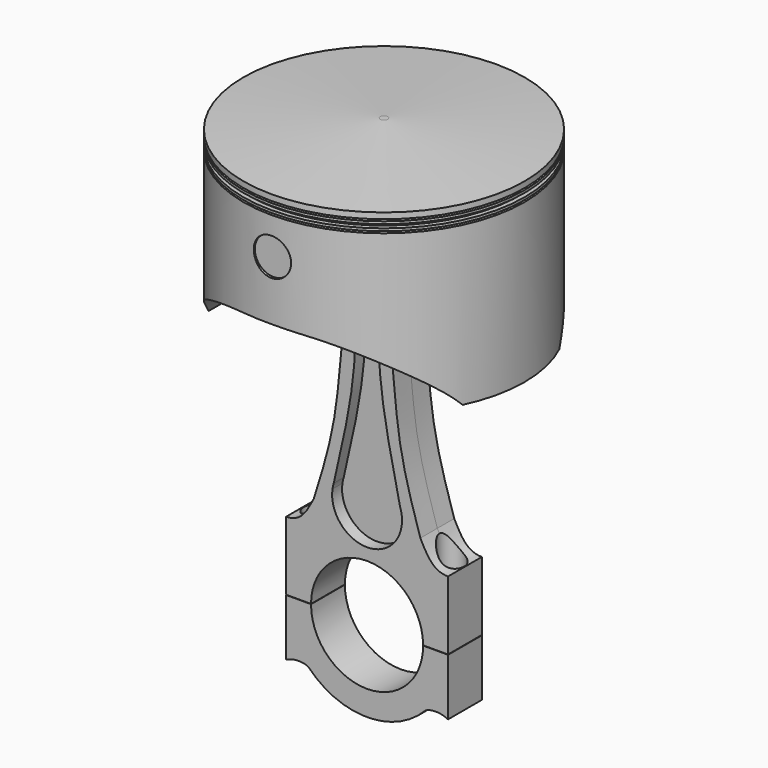
from build123d import *

# Parameters (mm, degrees)
F0_R           = 56.5
F1_DEPTH       = 75
F2_W           = 2
F2_H           = 0.75
F2_H_2         = 1.5
F4_SIZE2       = 4
F4_SIZE        = 55
F5_R           = 7.5
F6_DEPTH       = 100
F7_R           = 53.4676328736
F8_DEPTH       = 35.3
F10_END_RADIUS = 53.4676328736
F10_REACH      = 175.370336275
F11_END_RADIUS = 53.4676328736
F11_REACH      = 175.370336275
F12_W          = 30
F12_H          = 20
F13_DEPTH      = 65
F14_R          = 7.5
F15_DEPTH      = 8.5
F17_DEPTH      = 5
F19_DEPTH      = 5
F20_R          = 5
F21_DEPTH      = 95
F22_R          = 4
F23_DEPTH      = 12.5
F25_DEPTH      = 8.5
F26_R          = 4
F27_DEPTH      = 25
F28_R          = 7.5
F29_DEPTH      = 55.5


with BuildPart() as f1:
    # F0 (on Top) → F1 (new body)
    with BuildSketch(Plane.XY):
        Circle(F0_R)
    extrude(amount=F1_DEPTH)

    # F2 (on Front) → F3 (revolve, cut)
    with BuildSketch(Plane.XZ):
        with Locations((-55.6016643415, 68.2410276427)):
            Rectangle(F2_W, F2_H)
        with Locations((-55.6016643415, 66.1160276427)):
            Rectangle(F2_W, F2_H_2)
        with Locations((-55.6016643415, 63.9910276427)):
            Rectangle(F2_W, F2_H)
    revolve(axis=Axis((0, 0, 69.4315228611), (0, 0, 1)), mode=Mode.SUBTRACT)

    # F4
    f4_edges = [f1.edges().sort_by_distance(p)[0] for p in [
        (-56.5, 0, 75),
    ]]
    f4_side = f1.faces().sort_by_distance((0, 0, 75))[0]
    chamfer(f4_edges, length=F4_SIZE, length2=F4_SIZE2, reference=f4_side)

    # F5 (on Front) → F6 (cut, symmetric)
    with BuildSketch(Plane.XZ):
        with BuildLine():
            add(Edge.make_bspline(
                [(-51.0292984545, 0), (-46.6092862189, 10.918459855), (-25.7763816649, 24.8136985352), (-8.5923508332, 24.892498466), (0, 25.0624939799)],
                knots=[0, 0, 0, 0, 0.5341855486, 1, 1, 1, 1], degree=3))
            Line((-51.0292984545, 0), (51.0292984545, 0))
            add(Edge.make_bspline(
                [(51.0292984545, 0), (46.6092862189, 10.918459855), (25.7763816649, 24.8136985352), (8.5923508332, 24.892498466), (0, 25.0624939799)],
                knots=[0, 0, 0, 0, 0.5341855486, 1, 1, 1, 1], degree=3))
        make_face()
        with Locations((0, 48.8531067967)):
            Circle(F5_R)
    extrude(amount=F6_DEPTH, both=True, mode=Mode.SUBTRACT)

    # F7 (on face) → F8 (cut)
    with BuildSketch(Plane(origin=(0, 0, 0), x_dir=(1, 0, 0), z_dir=(0, 0, -1))):
        Circle(F7_R)
    extrude(amount=-F8_DEPTH, mode=Mode.SUBTRACT)

    f10_end = (Plane(origin=(0, 0, 17.65), x_dir=(-1, 0, 0), z_dir=(0, 0, -1)) * Cylinder(F10_END_RADIUS, 703.8015744111, mode=Mode.PRIVATE)).faces().sort_by_distance((-53.4676328736, 0, 17.65))[0]
    # F9 (on Front) → F10 (cut, up to the whole of a round face its end follows)
    with BuildSketch(Plane.XZ):
        with BuildLine():
            add(Edge.make_bspline(
                [(-32.6388143003, 57.5392916799), (-22.6882942127, 54.6689458554), (-14.6401413867, 36.5744103857), (-4.1431767228, 35.6272064229), (0, 34.9726118147)],
                knots=[0, 0, 0, 0, 0.5915213849, 1, 1, 1, 1], degree=3))
            add(Edge.make_bspline(
                [(-32.6388143003, 57.5392916799), (-38.0470310089, 58.2486421595), (-54.0857522846, 60.3523068689), (-52.0901718983, 24.0567715609), (-50.7674962282, 0)],
                knots=[0, 0, 0, 0, 0.3371974995, 1, 1, 1, 1], degree=3))
            Line((-50.7674962282, 0), (50.7674962282, 0))
            add(Edge.make_bspline(
                [(32.6388143003, 57.5392916799), (38.0470310089, 58.2486421595), (54.0857522846, 60.3523068689), (52.0901718983, 24.0567715609), (50.7674962282, 0)],
                knots=[0, 0, 0, 0, 0.3371974995, 1, 1, 1, 1], degree=3))
            add(Edge.make_bspline(
                [(32.6388143003, 57.5392916799), (22.6882942127, 54.6689458554), (14.6401413867, 36.5744103857), (4.1431767228, 35.6272064229), (0, 34.9726118147)],
                knots=[0, 0, 0, 0, 0.5915213849, 1, 1, 1, 1], degree=3))
        make_face()
    f10_long = extrude(amount=-F10_REACH, mode=Mode.PRIVATE)
    add(split(f10_long, bisect_by=f10_end, keep=Keep.BOTTOM, mode=Mode.PRIVATE), mode=Mode.SUBTRACT)

    f11_end = (Plane(origin=(0, 0, 29.0760973469), x_dir=(-1, 0, 0), z_dir=(0, 0, -1)) * Cylinder(F11_END_RADIUS, 703.8015744111, mode=Mode.PRIVATE)).faces().sort_by_distance((-53.4676328736, 0, 29.0760973469))[0]
    # F9 (on Front) → F11 (cut, up to the whole of a round face its end follows)
    with BuildSketch(Plane.XZ):
        with BuildLine():
            add(Edge.make_bspline(
                [(-32.6388143003, 57.5392916799), (-22.6882942127, 54.6689458554), (-14.6401413867, 36.5744103857), (-4.1431767228, 35.6272064229), (0, 34.9726118147)],
                knots=[0, 0, 0, 0, 0.5915213849, 1, 1, 1, 1], degree=3))
            add(Edge.make_bspline(
                [(-32.6388143003, 57.5392916799), (-38.0470310089, 58.2486421595), (-54.0857522846, 60.3523068689), (-52.0901718983, 24.0567715609), (-50.7674962282, 0)],
                knots=[0, 0, 0, 0, 0.3371974995, 1, 1, 1, 1], degree=3))
            Line((-50.7674962282, 0), (50.7674962282, 0))
            add(Edge.make_bspline(
                [(32.6388143003, 57.5392916799), (38.0470310089, 58.2486421595), (54.0857522846, 60.3523068689), (52.0901718983, 24.0567715609), (50.7674962282, 0)],
                knots=[0, 0, 0, 0, 0.3371974995, 1, 1, 1, 1], degree=3))
            add(Edge.make_bspline(
                [(32.6388143003, 57.5392916799), (22.6882942127, 54.6689458554), (14.6401413867, 36.5744103857), (4.1431767228, 35.6272064229), (0, 34.9726118147)],
                knots=[0, 0, 0, 0, 0.5915213849, 1, 1, 1, 1], degree=3))
        make_face()
    f11_long = extrude(amount=F11_REACH, mode=Mode.PRIVATE)
    add(split(f11_long, bisect_by=f11_end, keep=Keep.BOTTOM, mode=Mode.PRIVATE), mode=Mode.SUBTRACT)

    # F12 (on Top) → F13 (cut)
    with BuildSketch(Plane.XY):
        Rectangle(F12_W, F12_H)
    extrude(amount=F13_DEPTH, mode=Mode.SUBTRACT)


with BuildPart() as f15:
    # F14 (on Front) → F15 (new body, symmetric)
    with BuildSketch(Plane.XZ):
        with BuildLine():
            ThreePointArc((10.8046398623, 43.8526791523), (11.6973432528, 46.3956778919), (12, 49.073766917))
            ThreePointArc((12, 49.073766917), (-2.6780890251, 60.7711101698), (-10.8046398623, 43.8526791523))
            ThreePointArc((-10.8046398623, 43.8526791523), (0, 37.073766917), (10.8046398623, 43.8526791523))
        make_face()
        with Locations((0, 49.073766917)):
            Circle(F14_R, mode=Mode.SUBTRACT)
        with BuildLine():
            ThreePointArc((10.8046398623, 43.8526791523), (0, 37.073766917), (-10.8046398623, 43.8526791523))
            add(Edge.make_bspline(
                [(-10.8046398623, 43.8526791523), (-6.6073371508, 29.876045462), (-11.6452181528, -22.4009585178), (-13.7522928583, -39.2763094341), (-21.4106692265, -63.1426867915)],
                knots=[0, 0, 0, 0, 0.4754213594, 0.8884561444, 0.8884561444, 0.8884561444, 0.8884561444], degree=3))
            add(Edge.make_bspline(
                [(-21.4106692265, -63.1426867915), (-23.478884444, -69.5880222602), (-26.0341990895, -77.2018147862), (-29.2206345742, -86.4503130351)],
                knots=[0.8884561444, 0.8884561444, 0.8884561444, 0.8884561444, 1, 1, 1, 1], degree=3))
            ThreePointArc((-29.2206345742, -86.4503130351), (0, -68.1772071123), (29.2206345742, -86.4503130351))
            add(Edge.make_bspline(
                [(21.4106692265, -63.1426867915), (23.478884444, -69.5880222602), (26.0341990895, -77.2018147862), (29.2206345742, -86.4503130351)],
                knots=[0.8884561444, 0.8884561444, 0.8884561444, 0.8884561444, 1, 1, 1, 1], degree=3))
            add(Edge.make_bspline(
                [(10.8046398623, 43.8526791523), (6.6073371508, 29.876045462), (11.6452181528, -22.4009585178), (13.7522928583, -39.2763094341), (21.4106692265, -63.1426867915)],
                knots=[0, 0, 0, 0, 0.4754213594, 0.8884561444, 0.8884561444, 0.8884561444, 0.8884561444], degree=3))
        make_face()
        with BuildLine():
            add(Edge.make_bspline(
                [(-21.4106692265, -63.1426867915), (-23.478884444, -69.5880222602), (-26.0341990895, -77.2018147862), (-29.2206345742, -86.4503130351)],
                knots=[0.8884561444, 0.8884561444, 0.8884561444, 0.8884561444, 1, 1, 1, 1], degree=3))
            add(Edge.make_bspline(
                [(-32.5, -73.0932280421), (-26.3745859265, -73.0932280421), (-24.0367911756, -68.1578814983), (-21.4106692265, -63.1426867915)],
                knots=[0, 0, 0, 0, 14.8992123344, 14.8992123344, 14.8992123344, 14.8992123344], degree=3))
            Line((-32.5, -73.0932280421), (-32.5, -100.6772071123))
            ThreePointArc((-32.5, -100.6772071123), (-31.6695486521, -93.3772284706), (-29.2206345742, -86.4503130351))
        make_face()
        with BuildLine():
            add(Edge.make_bspline(
                [(32.5, -73.0932280421), (26.3745859265, -73.0932280421), (24.0367911756, -68.1578814983), (21.4106692265, -63.1426867915)],
                knots=[0, 0, 0, 0, 14.8992123344, 14.8992123344, 14.8992123344, 14.8992123344], degree=3))
            add(Edge.make_bspline(
                [(21.4106692265, -63.1426867915), (23.478884444, -69.5880222602), (26.0341990895, -77.2018147862), (29.2206345742, -86.4503130351)],
                knots=[0.8884561444, 0.8884561444, 0.8884561444, 0.8884561444, 1, 1, 1, 1], degree=3))
            ThreePointArc((29.2206345742, -86.4503130351), (31.6695486521, -93.3772284706), (32.5, -100.6772071123))
            Line((32.5, -100.6772071123), (32.5, -73.0932280421))
        make_face()
        with BuildLine():
            ThreePointArc((29.2206345742, -86.4503130351), (0, -68.1772071123), (-29.2206345742, -86.4503130351))
            ThreePointArc((-29.2206345742, -86.4503130351), (-31.6695486521, -93.3772284706), (-32.5, -100.6772071123))
            Line((-32.5, -100.6772071123), (-22.5, -100.6772071123))
            ThreePointArc((-22.5, -100.6772071123), (0, -78.1772071123), (22.5, -100.6772071123))
            Line((22.5, -100.6772071123), (32.5, -100.6772071123))
            ThreePointArc((32.5, -100.6772071123), (31.6695486521, -93.3772284706), (29.2206345742, -86.4503130351))
        make_face()
    extrude(amount=F15_DEPTH, both=True)

    # F16 (on face) → F17 (cut)
    with BuildSketch(Plane.XZ.offset(8.5)):
        with BuildLine():
            add(Edge.make_bspline(
                [(13.2256781798, -54.5839784182), (10.2358765284, -41.272635804), (4.8272921937, -16.567844843), (4.4394775777, 2.0371307447), (4.2555062992, 10.7180611238)],
                knots=[0.0423968026, 0.0423968026, 0.0423968026, 0.0423968026, 0.5531914948, 1, 1, 1, 1], degree=3))
            ThreePointArc((4.2555062992, 10.7180611238), (0.2066547481, 16.1602928365), (-4.3365096734, 11.1233550825))
            add(Edge.make_bspline(
                [(-13.3671997476, -55.0014076796), (-10.3278424538, -41.9185277358), (-4.74044347, -17.4056606078), (-4.4641681007, 2.0087009883), (-4.3365096734, 11.1233550825)],
                knots=[0.0296485709, 0.0296485709, 0.0296485709, 0.0296485709, 0.5444008536, 1, 1, 1, 1], degree=3))
            add(Edge.make_bspline(
                [(-13.8928588849, -57.26257095), (-13.7175699845, -56.5087594933), (-13.5422598752, -55.754952068), (-13.3671997476, -55.0014076796)],
                knots=[0, 0, 0, 0, 0.0296485709, 0.0296485709, 0.0296485709, 0.0296485709], degree=3))
            ThreePointArc((-13.8928588849, -57.26257095), (-0.3213398083, -73.3384730153), (13.9715628795, -57.9004132273))
            add(Edge.make_bspline(
                [(13.9715628795, -57.9004132273), (13.7227171973, -56.794625448), (13.4738366524, -55.688841829), (13.2256781798, -54.5839784182)],
                knots=[0, 0, 0, 0, 0.0423968026, 0.0423968026, 0.0423968026, 0.0423968026], degree=3))
        make_face()
        with BuildLine():
            ThreePointArc((13.9715628795, -57.9004132273), (13.699349082, -56.2195414091), (13.2256781798, -54.5839784182))
            add(Edge.make_bspline(
                [(13.9715628795, -57.9004132273), (13.7227171973, -56.794625448), (13.4738366524, -55.688841829), (13.2256781798, -54.5839784182)],
                knots=[0, 0, 0, 0, 0.0423968026, 0.0423968026, 0.0423968026, 0.0423968026], degree=3))
        make_face()
        with BuildLine():
            add(Edge.make_bspline(
                [(-13.8928588849, -57.26257095), (-13.7175699845, -56.5087594933), (-13.5422598752, -55.754952068), (-13.3671997476, -55.0014076796)],
                knots=[0, 0, 0, 0, 0.0296485709, 0.0296485709, 0.0296485709, 0.0296485709], degree=3))
            ThreePointArc((-13.3671997476, -55.0014076796), (-13.6768385965, -56.1211074266), (-13.8928588849, -57.26257095))
        make_face()
    extrude(amount=-F17_DEPTH, mode=Mode.SUBTRACT)

    # F18 (on face) → F19 (cut)
    with BuildSketch(Plane(origin=(0, 8.5, 0), x_dir=(-1, 0, 0), z_dir=(0, 1, 0))):
        with BuildLine():
            add(Edge.make_bspline(
                [(13.1423263541, -55.4686981502), (10.1525247027, -42.157355536), (4.7439403679, -17.452564575), (4.3561257519, 1.1524110127), (4.1721544735, 9.8333413918)],
                knots=[0.0423968026, 0.0423968026, 0.0423968026, 0.0423968026, 0.5531914948, 1, 1, 1, 1], degree=3))
            ThreePointArc((4.1721544735, 9.8333413918), (0.1233029223, 15.2755731045), (-4.4198614992, 10.2386353505))
            add(Edge.make_bspline(
                [(-13.4505515734, -55.8861274116), (-10.4111942796, -42.8032474678), (-4.8237952957, -18.2903803398), (-4.5475199264, 1.1239812563), (-4.4198614992, 10.2386353505)],
                knots=[0.0296485709, 0.0296485709, 0.0296485709, 0.0296485709, 0.5444008536, 1, 1, 1, 1], degree=3))
            add(Edge.make_bspline(
                [(-13.9762107106, -58.1472906819), (-13.8009218103, -57.3934792253), (-13.625611701, -56.6396717999), (-13.4505515734, -55.8861274116)],
                knots=[0, 0, 0, 0, 0.0296485709, 0.0296485709, 0.0296485709, 0.0296485709], degree=3))
            ThreePointArc((-13.9762107106, -58.1472906819), (-0.4046916341, -74.2231927473), (13.8882110538, -58.7851329593))
            add(Edge.make_bspline(
                [(13.8882110538, -58.7851329593), (13.6393653715, -57.67934518), (13.3904848266, -56.573561561), (13.1423263541, -55.4686981502)],
                knots=[0, 0, 0, 0, 0.0423968026, 0.0423968026, 0.0423968026, 0.0423968026], degree=3))
        make_face()
    extrude(amount=-F19_DEPTH, mode=Mode.SUBTRACT)

    # F20 (on Top) → F21 (cut)
    with BuildSketch(Plane.XY):
        with Locations((-27.2349342704, 0)):
            Circle(F20_R)
        with Locations((27.2349342704, 0)):
            Circle(F20_R)
    extrude(amount=-F21_DEPTH, mode=Mode.SUBTRACT)

    # F22 (on face) → F23 (cut, symmetric)
    with BuildSketch(Plane(origin=(0, 0, -100.6772071123), x_dir=(1, 0, 0), z_dir=(0, 0, -1))):
        with Locations((-27.5008101016, 0)):
            Circle(F22_R)
        with Locations((27.5008101016, 0)):
            Circle(F22_R)
    extrude(amount=F23_DEPTH, both=True, mode=Mode.SUBTRACT)


with BuildPart() as f25:
    # F24 (on Front) → F25 (new body, symmetric)
    with BuildSketch(Plane.XZ):
        with BuildLine():
            ThreePointArc((22.4996449488, -100.7931661889), (0, -123.4195670485), (-22.4996449488, -100.7931661889))
            Line((-22.4996449488, -100.7931661889), (-32.4997541963, -100.7931661889))
            Line((-32.4997541963, -100.7931661889), (-32.4997541963, -101.0459679082))
            Line((-32.4997541963, -101.0459679082), (-32.4997541963, -123.6481294036))
            add(Edge.make_bspline(
                [(-32.4997541963, -123.6481294036), (-28.9459917694, -121.7721700668), (-24.3484551304, -122.4463580951), (-23.2306360927, -123.6481294036)],
                knots=[0, 0, 0, 0, 9.2691181036, 9.2691181036, 9.2691181036, 9.2691181036], degree=3))
            ThreePointArc((-23.2306360927, -123.6481294036), (0, -133.4195670485), (23.2306360927, -123.6481294036))
            add(Edge.make_bspline(
                [(32.4997541963, -123.6481294036), (28.9459917694, -121.7721700668), (24.3484551304, -122.4463580951), (23.2306360927, -123.6481294036)],
                knots=[0, 0, 0, 0, 9.2691181036, 9.2691181036, 9.2691181036, 9.2691181036], degree=3))
            Line((32.4997541963, -123.6481294036), (32.4997541963, -101.0459679082))
            Line((32.4997541963, -101.0459679082), (32.4997541963, -100.7931661889))
            Line((32.4997541963, -100.7931661889), (22.4996449488, -100.7931661889))
        make_face()
        with BuildLine():
            Line((-32.4997541963, -101.0459679082), (-32.4997541963, -100.7931661889))
            ThreePointArc((-32.4997541963, -100.7931661889), (-32.5, -100.9195670485), (-32.4997541963, -101.0459679082))
        make_face()
        with BuildLine():
            ThreePointArc((32.4997541963, -101.0459679082), (32.5, -100.9195670485), (32.4997541963, -100.7931661889))
            Line((32.4997541963, -100.7931661889), (32.4997541963, -101.0459679082))
        make_face()
    extrude(amount=F25_DEPTH, both=True)

    # F26 (on face) → F27 (cut)
    with BuildSketch(Plane.XY.offset(-100.7931661889)):
        with Locations((-27.4996995726, 0)):
            Circle(F26_R)
        with Locations((27.4996995726, 0)):
            Circle(F26_R)
    extrude(amount=-F27_DEPTH, mode=Mode.SUBTRACT)


with BuildPart() as f29:
    # F28 (on Front) → F29 (new body, symmetric)
    with BuildSketch(Plane.XZ):
        with Locations((0, 48.7527400255)):
            Circle(F28_R)
    extrude(amount=F29_DEPTH, both=True)


solid = Compound([f1.part, f15.part, f25.part, f29.part])
